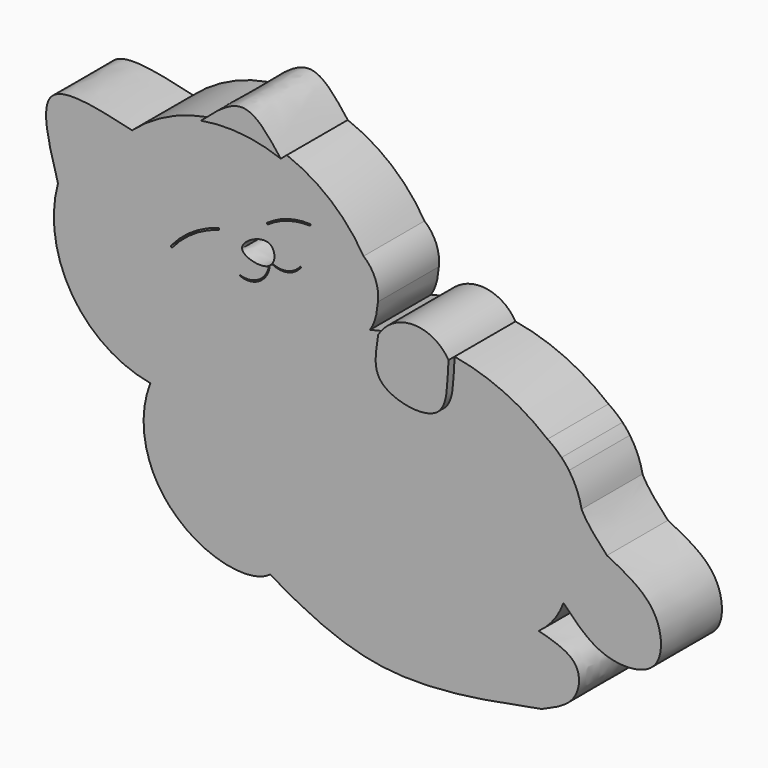
from build123d import *

# Parameters (mm, degrees)
F1_DEPTH = 12.7
F2_DEPTH = 13.97


with BuildPart() as f1:
    # F0 (on Front) → F1 (new body)
    with BuildSketch(Plane.XZ):
        with BuildLine():
            add(Edge.make_bspline(
                [(59.1061716019, -4.2043621835), (58.3953510036, -3.510707878), (57.5753379472, -2.8959754481), (56.7613643321, -2.276264629)],
                knots=[0.8131179307, 0.8131179307, 0.8131179307, 0.8131179307, 1, 1, 1, 1], degree=3))
            ThreePointArc((56.7613643321, -2.276264629), (49.4791419592, 2.277986697), (41.2694336671, 4.8023990217))
            add(Edge.make_bspline(
                [(29.5313251719, 4.6794850926), (29.1414100604, 1.9221812865), (27.9308180864, -3.4101647296), (41.8323133175, -5.906469104), (40.9844336777, 1.749254351), (41.2694336671, 4.8023990217)],
                knots=[0, 0, 0, 0, 0.1570486005, 0.3364582627, 0.510386675, 0.510386675, 0.510386675, 0.510386675], degree=3))
            ThreePointArc((29.5313251719, 4.6794850926), (28.3420191938, 4.4292771407), (27.1627145152, 4.1355200917))
            add(Edge.make_bspline(
                [(28.4860077977, 8.6753729454), (28.3390382985, 7.2053221936), (28.1920687992, 5.7352714419), (27.1627145152, 4.1355200917)],
                knots=[0, 0, 0, 0, 0.3706313521, 0.3706313521, 0.3706313521, 0.3706313521], degree=3))
            ThreePointArc((28.4860077977, 8.6753729454), (28.0391099274, 11.9438353715), (26.0936398085, 14.6079882112))
            ThreePointArc((26.0936398085, 14.6079882112), (20.5948318097, 21.0205895609), (13.2967198545, 25.2745180236))
            ThreePointArc((13.2967198545, 25.2745180236), (6.7327034589, 26.7945457305), (0, 26.5347388693))
            ThreePointArc((0, 26.5347388693), (-6.6651341425, 24.4005933469), (-12.4945323914, 20.5280352384))
            add(Edge.make_bspline(
                [(-24.8554814607, 8.7302317843), (-26.3582845919, 13.9286221672), (-29.4227370154, 24.5289594145), (-18.2090454728, 21.878641168), (-12.4945323914, 20.5280352384)],
                knots=[0, 0, 0, 0, 0.4903985847, 1, 1, 1, 1], degree=3))
            ThreePointArc((-24.8554814607, 8.7302317843), (-22.5230177273, -6.8283307763), (-9.4597768039, -15.5953709036))
            ThreePointArc((-9.4597768039, -15.5953709036), (-10.5806893026, -21.3422223383), (-9.6007177755, -27.1147782755))
            add(Edge.make_bspline(
                [(-9.6007177755, -27.1147782755), (-8.5647365316, -29.5135595921), (-7.0556106981, -31.9100860204), (-5.0480626523, -33.7880067527)],
                knots=[0.2832101572, 0.2832101572, 0.2832101572, 0.2832101572, 0.3975900868, 0.3975900868, 0.3975900868, 0.3975900868], degree=3))
            add(Edge.make_bspline(
                [(-5.0480626523, -33.7880067527), (-0.3306821613, -38.2007861357), (7.1388179474, -39.7499994998), (10.5236132672, -37.1664466075)],
                knots=[0.3975900868, 0.3975900868, 0.3975900868, 0.3975900868, 0.6663625578, 0.6663625578, 0.6663625578, 0.6663625578], degree=3))
            add(Edge.make_bspline(
                [(55.5000454187, -42.2575362027), (45.9227569206, -44.1077921969), (29.534223499, -47.2739265579), (16.0171883325, -40.4395783324), (10.5236132672, -37.1664466075)],
                knots=[0, 0, 0, 0, 0.5131163927, 0.8780381998, 0.8780381998, 0.8780381998, 0.8780381998], degree=3))
            Line((55.5000454187, -42.2575362027), (55.6802488863, -42.2575362027))
            add(Edge.make_bspline(
                [(55.6802488863, -42.2575362027), (57.8649319172, -41.3421819694), (61.933363626, -39.6375611457), (62.5441736967, -32.9275500123), (57.8690689466, -31.5816055418), (55.2858944788, -30.8987696483)],
                knots=[0, 0, 0, 0, 0.3430550385, 0.6388551459, 0.9830517596, 0.9830517596, 0.9830517596, 0.9830517596], degree=3))
            ThreePointArc((55.2858944788, -30.8987696483), (57.774796408, -28.4914379114), (59.4194548829, -25.4443118219))
            add(Edge.make_bspline(
                [(59.4194548829, -25.4443118219), (61.5668623777, -27.6961704589), (65.7267940312, -32.0584435934), (76.3421290349, -31.3246256264), (75.736400422, -20.6626458704), (69.8191952556, -17.7023380158), (66.6726157069, -16.128141433)],
                knots=[0, 0, 0, 0, 0.2566051025, 0.4970922803, 0.7325698364, 1, 1, 1, 1], degree=3))
            add(Edge.make_bspline(
                [(66.6726157069, -16.128141433), (65.0447675311, -14.3832892567), (63.4100748942, -12.6418994745), (62.438506633, -10.718587786)],
                knots=[0, 0, 0, 0, 0.3651247136, 0.3651247136, 0.3651247136, 0.3651247136], degree=3))
            add(Edge.make_bspline(
                [(62.438506633, -10.718587786), (61.5739147936, -9.0070460887), (61.2344575356, -7.1514386813), (60.3355277859, -5.7014262697)],
                knots=[0.3651247136, 0.3651247136, 0.3651247136, 0.3651247136, 0.6900466571, 0.6900466571, 0.6900466571, 0.6900466571], degree=3))
            ThreePointArc((60.3355277859, -5.7014262697), (59.7492819423, -4.929546288), (59.1061716019, -4.2043621835))
        make_face()
        with BuildLine():
            ThreePointArc((-5.9990617447, 5.7310229167), (-2.4740959169, 8.8804908185), (1.8180131447, 10.8609786257))
            ThreePointArc((1.8180131447, 10.8609786257), (2.0089152962, 10.7924724578), (1.9302222129, 10.60553898))
            ThreePointArc((1.9302222129, 10.60553898), (-2.3105141336, 8.6258077241), (-5.79586206, 5.5024232715))
            ThreePointArc((-5.79586206, 5.5024232715), (-5.9682689093, 5.5537835324), (-5.9990617447, 5.7310229167))
        make_face(mode=Mode.SUBTRACT)
        with BuildLine():
            add(Edge.make_bspline(
                [(10.3070973536, 8.028651153), (8.8878162788, 7.2321778462), (5.9498321238, 8.001992808), (5.8378027752, 9.1516999528)],
                knots=[0.6626685216, 0.6626685216, 0.6626685216, 0.6626685216, 1, 1, 1, 1], degree=3))
            add(Edge.make_bspline(
                [(5.8378027752, 9.1516999528), (5.7188398768, 10.3725630212), (10.8860088037, 13.1505736904), (11.5140866455, 9.5170493858), (10.9034565546, 8.586031805)],
                knots=[0, 0, 0, 0, 0.3582090845, 0.6033763358, 0.6033763358, 0.6033763358, 0.6033763358], degree=3))
            ThreePointArc((10.9034565546, 8.586031805), (13.3764537584, 8.2942058615), (15.4947527988, 9.6032844405))
            ThreePointArc((15.4947527988, 9.6032844405), (15.6035241906, 9.6130970285), (15.6345004432, 9.5083689314))
            ThreePointArc((15.6345004432, 9.5083689314), (13.4210728493, 8.1059221778), (10.8274193225, 8.4788564786))
            add(Edge.make_bspline(
                [(10.8274193225, 8.4788564786), (10.7248464569, 8.3450423002), (10.6024036816, 8.2251174819), (10.4596894234, 8.1246141344)],
                knots=[0.6130144256, 0.6130144256, 0.6130144256, 0.6130144256, 0.6500567437, 0.6500567437, 0.6500567437, 0.6500567437], degree=3))
            ThreePointArc((10.4596894234, 8.1246141344), (8.7756345565, 5.3284277831), (5.5296770297, 4.9842495724))
            ThreePointArc((5.5296770297, 4.9842495724), (5.4924518419, 5.0703022397), (5.5651250629, 5.1295422522))
            ThreePointArc((5.5651250629, 5.1295422522), (8.601479146, 5.4907773493), (10.3070973536, 8.028651153))
        make_face(mode=Mode.SUBTRACT)
        with BuildLine():
            ThreePointArc((9.9886422977, 14.2604736611), (13.3617809031, 15.9412203037), (17.0977395028, 16.4367873222))
            ThreePointArc((17.0977395028, 16.4367873222), (17.2505331806, 16.3157218017), (17.1331140203, 16.16010847))
            ThreePointArc((17.1331140203, 16.16010847), (13.4617569094, 15.6841100404), (10.1337671161, 14.0624067764))
            ThreePointArc((10.1337671161, 14.0624067764), (9.9877830492, 14.1076437209), (9.9886422977, 14.2604736611))
        make_face(mode=Mode.SUBTRACT)
        with BuildLine():
            ThreePointArc((59.1061716019, -4.2043621835), (57.9912746912, -3.1703780522), (56.7613643321, -2.276264629))
            add(Edge.make_bspline(
                [(59.1061716019, -4.2043621835), (58.3953510036, -3.510707878), (57.5753379472, -2.8959754481), (56.7613643321, -2.276264629)],
                knots=[0.8131179307, 0.8131179307, 0.8131179307, 0.8131179307, 1, 1, 1, 1], degree=3))
        make_face()
        with BuildLine():
            ThreePointArc((62.438506633, -10.718587786), (61.657325801, -8.0967052638), (60.3355277859, -5.7014262697))
            add(Edge.make_bspline(
                [(62.438506633, -10.718587786), (61.5739147936, -9.0070460887), (61.2344575356, -7.1514386813), (60.3355277859, -5.7014262697)],
                knots=[0.3651247136, 0.3651247136, 0.3651247136, 0.3651247136, 0.6900466571, 0.6900466571, 0.6900466571, 0.6900466571], degree=3))
        make_face()
        with BuildLine():
            ThreePointArc((-9.6007177755, -27.1147782755), (-7.7438934974, -30.7375888851), (-5.0480626523, -33.7880067527))
            add(Edge.make_bspline(
                [(-9.6007177755, -27.1147782755), (-8.5647365316, -29.5135595921), (-7.0556106981, -31.9100860204), (-5.0480626523, -33.7880067527)],
                knots=[0.2832101572, 0.2832101572, 0.2832101572, 0.2832101572, 0.3975900868, 0.3975900868, 0.3975900868, 0.3975900868], degree=3))
        make_face()
    extrude(amount=F1_DEPTH)

    # F0 (on Front) → F2 (join)
    with BuildSketch(Plane.XZ):
        with BuildLine():
            add(Edge.make_bspline(
                [(29.5313251719, 4.6794850926), (29.1414100604, 1.9221812865), (27.9308180864, -3.4101647296), (41.8323133175, -5.906469104), (40.9844336777, 1.749254351), (41.2694336671, 4.8023990217)],
                knots=[0, 0, 0, 0, 0.1570486005, 0.3364582627, 0.510386675, 0.510386675, 0.510386675, 0.510386675], degree=3))
            ThreePointArc((41.2694336671, 4.8023990217), (35.3652424418, 8.0964743323), (29.5313251719, 4.6794850926))
        make_face()
        with BuildLine():
            ThreePointArc((0, 26.5347388693), (6.7327034589, 26.7945457305), (13.2967198545, 25.2745180236))
            add(Edge.make_bspline(
                [(0, 26.5347388693), (2.4426200797, 28.7145279713), (7.327860239, 33.0741061753), (11.3070999826, 27.8743807408), (13.2967198545, 25.2745180236)],
                knots=[0, 0, 0, 0, 0.5, 1, 1, 1, 1], degree=3))
        make_face()
    extrude(amount=F2_DEPTH)


solid = f1.part
